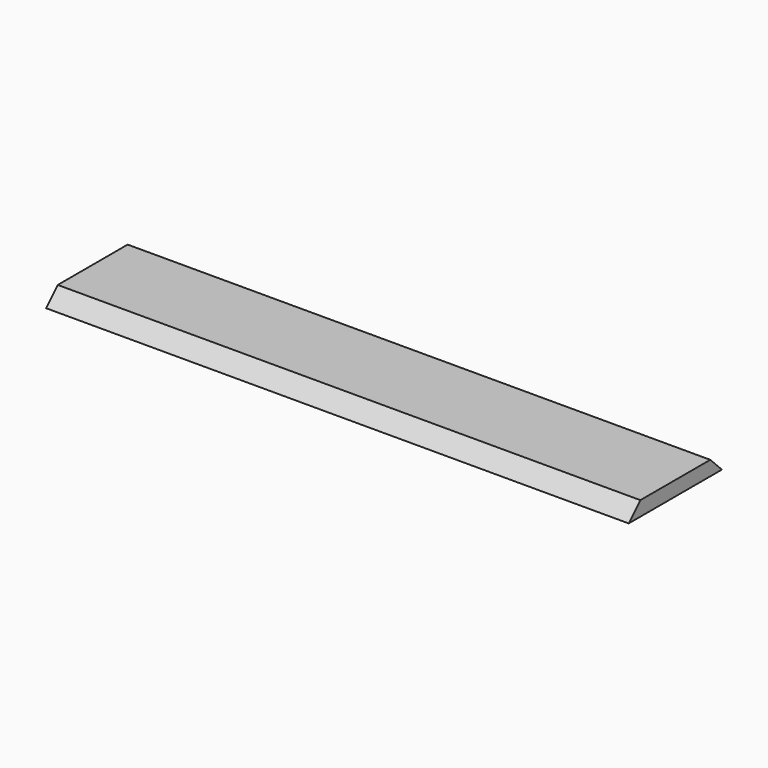
from build123d import *

# Parameters (mm, degrees)
F0_W     = 381
F0_H     = 76.2
F1_DEPTH = 9.525
F3_DEPTH = 381.001


# Not quite as in the source:
# - a length typed as a fraction of an inch, garbled in the dataset ("3 / 203.2 mm" for 3/8 in), is restored


with BuildPart() as f1:
    # F0 (on Top) → F1 (new body)
    with BuildSketch(Plane.XY):
        Rectangle(F0_W, F0_H)
    extrude(amount=F1_DEPTH)

    # F2 (on face) → F3 (cut, through all)
    with BuildSketch(Plane.YZ.offset(190.5)):
        Polygon((-42.2204956412, -2.0329502877), (-38.1, 0), (-28.575, 9.525), (-39.3758900464, 14.3782440573), align=None)
        Polygon((42.2204956412, -2.0329502877), (39.3758900464, 14.3782440573), (28.575, 9.525), (38.1, 0), align=None)
    extrude(amount=-F3_DEPTH, mode=Mode.SUBTRACT)


solid = f1.part
